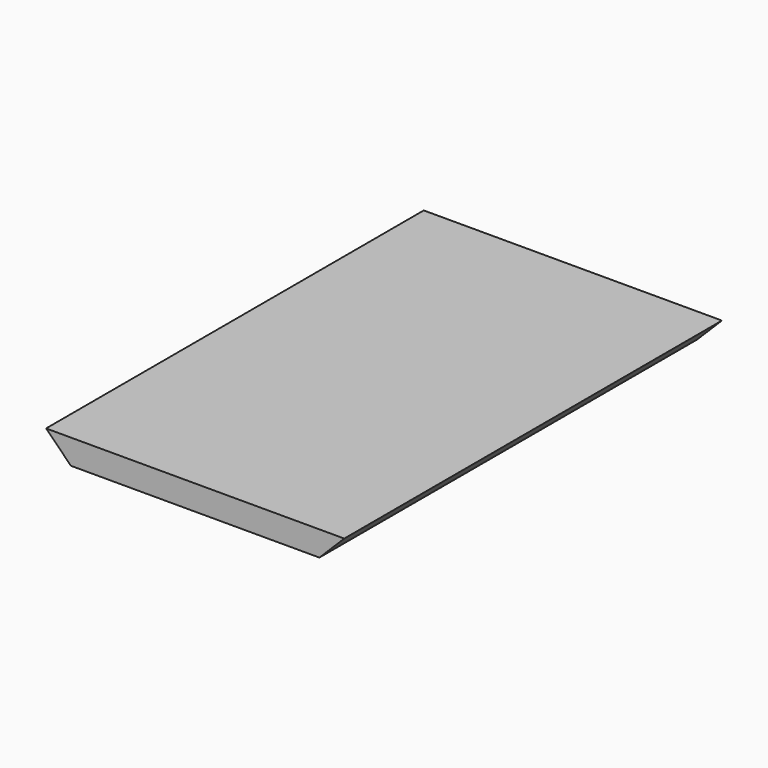
from build123d import *

# Parameters (mm, degrees)
F0_W     = 228.6
F0_H     = 361.95
F1_DEPTH = 19.05
F2_SIZE  = 19.04999


# Not quite as in the source:
# - a fillet or chamfer is up to 0.001 mm smaller than in the source, because OpenCascade refuses the exact size


with BuildPart() as f1:
    # F0 (on Top) → F1 (new body)
    with BuildSketch(Plane.XY):
        Rectangle(F0_W, F0_H)
    extrude(amount=F1_DEPTH)

    # F2 (size 19.05 in the source; OpenCascade refuses exactly that, so slightly less here)
    f2_edges = [f1.edges().sort_by_distance(p)[0] for p in [
        (114.3, 0, 0),
        (-114.3, 0, 0),
    ]]
    chamfer(f2_edges, length=F2_SIZE)


solid = f1.part
